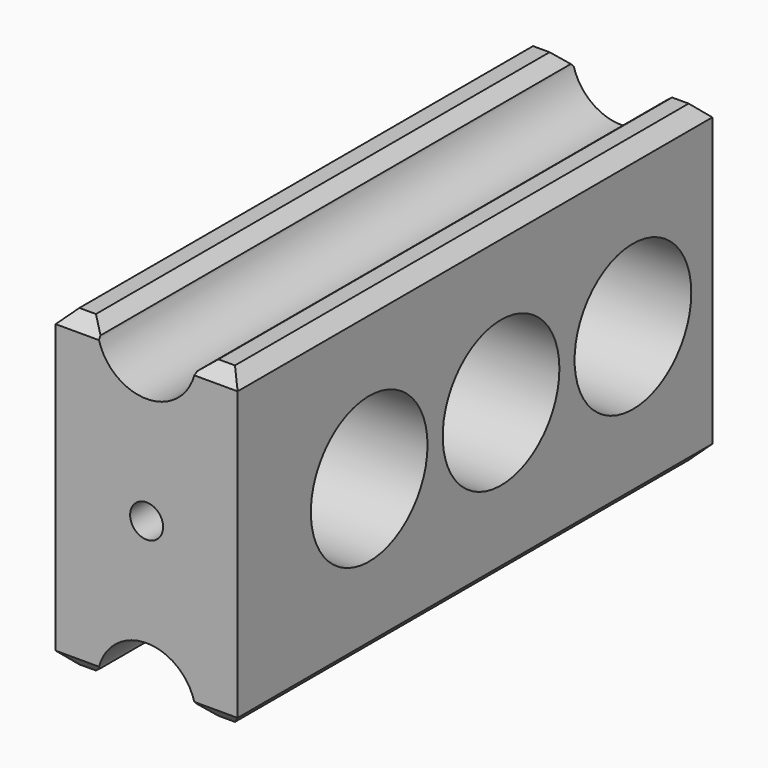
from build123d import *

# Parameters (mm, degrees)
F0_W        = 35.052
F0_H        = 60.452
F1_DEPTH    = 114.3
F2_R        = 14.0462
F3_DEPTH    = 35.053
F4_R        = 3.175
F5_DEPTH    = 25.4
F6_R        = 9.525
F7_DEPTH    = 114.301
F8_T1_DEPTH = 21.0651495789
F8_T3_DEPTH = 127.3641495789
F8_T5_DEPTH = 126.047561274
F8_T7_DEPTH = 21.0651495789


# Not quite as in the source:
# - a fillet or chamfer that OpenCascade refuses, or shapes differently, is made with other operations: its cross-section is extruded or revolved along the edge and cut away or added


with BuildPart() as f1:
    # F0 (on Front) → F1 (new body)
    with BuildSketch(Plane.XZ):
        Rectangle(F0_W, F0_H)
    extrude(amount=F1_DEPTH)

    # F2 (on face) → F3 (cut, through all)
    with BuildSketch(Plane.YZ.offset(17.526)):
        with Locations((-19.1262, 0)):
            Circle(F2_R)
        with Locations((-50.8762, 0)):
            Circle(F2_R)
        with Locations((-82.6262, 0)):
            Circle(F2_R)
    extrude(amount=-F3_DEPTH, mode=Mode.SUBTRACT)

    # F4 (on face) → F5 (cut)
    with BuildSketch(Plane.XZ.offset(114.3)):
        Circle(F4_R)
    extrude(amount=-F5_DEPTH, mode=Mode.SUBTRACT)

    # F6 (on face) → F7 (cut, through all)
    with BuildSketch(Plane.XZ.offset(114.3)):
        with Locations((0, 30.226)):
            Circle(F6_R)
        with Locations((0, -30.226)):
            Circle(F6_R)
    extrude(amount=-F7_DEPTH, mode=Mode.SUBTRACT)

    # F8: chamfer of 2.54 on 16 edges, made by hand

    # F8_s2 → F8_t1 (cut)
    with BuildSketch(Plane.YZ.offset(-24.0580747894)):
        Polygon((-2.54, 30.226), (0, 27.686), (0, 30.226), align=None)
        Polygon((-111.76, 30.226), (-114.3, 27.686), (-114.3, 30.226), align=None)
        Polygon((0, -27.686), (-2.54, -30.226), (0, -30.226), align=None)
        Polygon((-114.3, -27.686), (-111.76, -30.226), (-114.3, -30.226), align=None)
    extrude(amount=F8_T1_DEPTH, mode=Mode.SUBTRACT)

    # F8_s4 → F8_t3 (cut)
    with BuildSketch(Plane.XZ.offset(-6.5320747894)):
        Polygon((-17.526, 27.686), (-14.986, 30.226), (-17.526, 30.226), align=None)
        Polygon((14.986, 30.226), (17.526, 27.686), (17.526, 30.226), align=None)
        Polygon((-17.526, -27.686), (-14.986, -30.226), (-17.526, -30.226), align=None)
        Polygon((17.526, -27.686), (14.986, -30.226), (17.526, -30.226), align=None)
    extrude(amount=F8_T3_DEPTH, mode=Mode.SUBTRACT)

    # F8_s6 → F8_t5 (cut)
    with BuildSketch(Plane.XZ.offset(-5.873780637)):
        with BuildLine():
            Line((-11.7946015193, 30.226), (-9.3115275153, 28.2207368421))
            ThreePointArc((-9.3115275153, 28.2207368421), (-9.4675743486, 29.181652858), (-9.525, 30.226))
            Line((-9.525, 30.226), (-11.7946015193, 30.226))
        make_face()
        with BuildLine():
            Line((9.3115275153, 28.2207368421), (11.7946015193, 30.226))
            Line((11.7946015193, 30.226), (9.525, 30.226))
            ThreePointArc((9.525, 30.226), (9.4675743486, 29.181652858), (9.3115275153, 28.2207368421))
        make_face()
        with BuildLine():
            Line((-11.7946015193, -30.226), (-9.3115275153, -28.2207368421))
            ThreePointArc((-9.3115275153, -28.2207368421), (-9.4675743486, -29.181652858), (-9.525, -30.226))
            Line((-9.525, -30.226), (-11.7946015193, -30.226))
        make_face()
        with BuildLine():
            Line((11.7946015193, -30.226), (9.3115275153, -28.2207368421))
            ThreePointArc((9.3115275153, -28.2207368421), (9.4675743486, -29.181652858), (9.525, -30.226))
            Line((9.525, -30.226), (11.7946015193, -30.226))
        make_face()
    extrude(amount=F8_T5_DEPTH, mode=Mode.SUBTRACT)

    # F8_s8 → F8_t7 (cut)
    with BuildSketch(Plane.YZ.offset(2.9929252106)):
        Polygon((0, 27.686), (-2.54, 30.226), (0, 30.226), align=None)
        Polygon((-114.3, 27.686), (-111.76, 30.226), (-114.3, 30.226), align=None)
        Polygon((0, -27.686), (-2.54, -30.226), (0, -30.226), align=None)
        Polygon((-114.3, -27.686), (-111.76, -30.226), (-114.3, -30.226), align=None)
    extrude(amount=F8_T7_DEPTH, mode=Mode.SUBTRACT)


solid = f1.part
